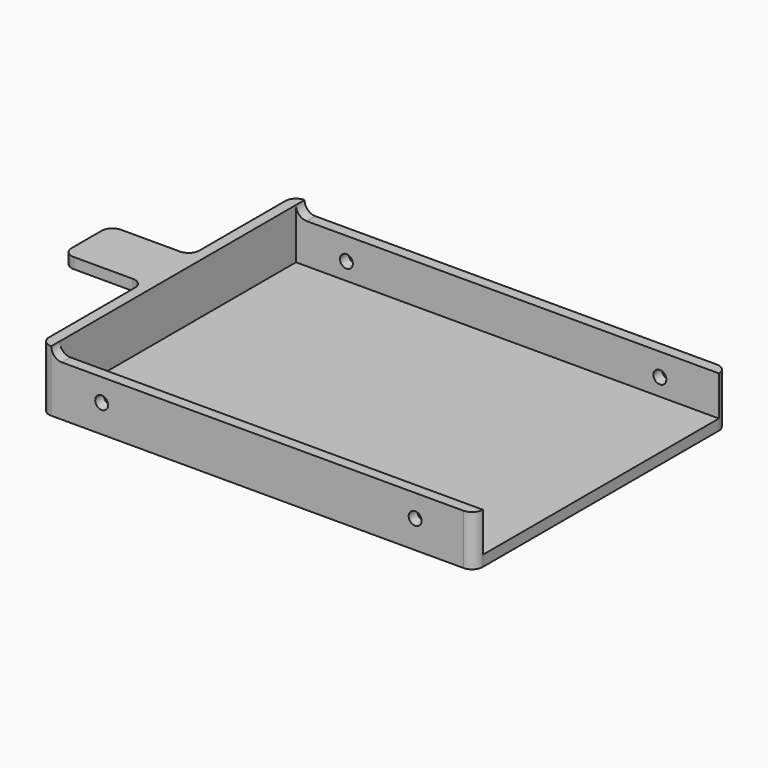
from build123d import *

# Parameters (mm, degrees)
F0_W     = 100.076
F0_H     = 2.54
F1_DEPTH = 11.938
F0_H_2   = 69.85
F2_DEPTH = 2.54
F4_DEPTH = 14.478
F5_W     = 13.97
F5_H     = 2.54
F6_DEPTH = 19.05
F7_R     = 2.5399
F3_R     = 1.524
F8_DEPTH = 76.2


# Not quite as in the source:
# - a fillet or chamfer is up to 0.001 mm smaller than in the source, because OpenCascade refuses the exact size


with BuildPart() as f1:
    # F0 (on Top) → F1 (new body)
    with BuildSketch(Plane.XY):
        with Locations((50.038, 71.12)):
            Rectangle(F0_W, F0_H)
    extrude(amount=F1_DEPTH)



with BuildPart() as f1b:
    # F0 (on Top) → F1, piece 2 (new body)
    with BuildSketch(Plane.XY):
        with Locations((50.038, -1.27)):
            Rectangle(F0_W, F0_H)
    extrude(amount=F1_DEPTH)


with BuildPart() as f1_1:
    add(f1.part)

    add(f1b.part)  # F2 merges F1b
    # F0 (on Top) → F2 (join)
    with BuildSketch(Plane.XY):
        with Locations((50.038, 34.925)):
            Rectangle(F0_W, F0_H_2)
    extrude(amount=F2_DEPTH)

    # F0 (on Top) → F4 (join)
    with BuildSketch(Plane.XY):
        Polygon((0, -2.54), (0, 0), (0, 69.85), (0, 72.39), (-2.54, 72.39), (-2.54, -2.54), align=None)
    extrude(amount=F4_DEPTH)

    # F5 (on face) → F6 (join)
    with BuildSketch(Plane(origin=(-2.54, 0, 0), x_dir=(0, -1, 0), z_dir=(-1, 0, 0))):
        with Locations((-34.925, 13.208)):
            Rectangle(F5_W, F5_H)
    extrude(amount=F6_DEPTH)

    # F7 (radius 2.54 in the source; OpenCascade refuses exactly that, so slightly less here)
    f7_edges = [f1_1.edges().sort_by_distance(p)[0] for p in [
        (-21.59, 27.94, 13.208),
        (-21.59, 41.91, 13.208),
        (-2.54, 41.91, 13.208),
        (-2.54, 27.94, 13.208),
        (-2.54, -2.54, 7.239),
        (100.076, -2.54, 5.969),
        (100.076, 72.39, 5.969),
        (-2.54, 72.39, 7.239),
        (0, 71.12, 11.938),
        (0, -1.27, 11.938),
        (-2.54, 34.925, 11.938),
    ]]
    fillet(f7_edges, radius=F7_R)

    # F3 (on face) → F8 (cut)
    with BuildSketch(Plane.XZ.offset(2.54)):
        with Locations((86.106, 6.604)):
            Circle(F3_R)
        with Locations((11.938, 6.604)):
            Circle(F3_R)
    extrude(amount=-F8_DEPTH, mode=Mode.SUBTRACT)


solid = f1_1.part
